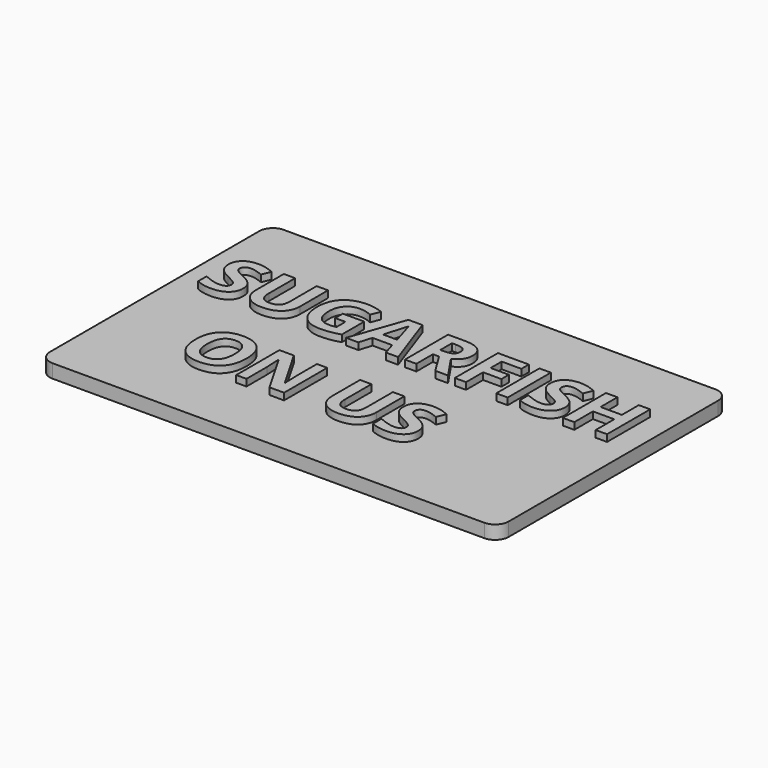
from build123d import *

# Parameters (mm, degrees)
F1_DEPTH     = 2.54
F2_TEXT_SIZE = 14.1111111111
F3_DEPTH     = 1.27


# Not quite as in the source:
# - Text() gives the source's letters only with a copy of the font that has no kerning and outlines rounded to 1/6400 em; it was checked with that copy


with BuildPart() as f1:
    # F0 (on Top) → F1 (new body)
    with BuildSketch(Plane.XY):
        with BuildLine():
            ThreePointArc((42.8625, 24.4475), (42.1185512242, 26.2435512242), (40.3225, 26.9875))
            Line((40.3225, 26.9875), (-40.3225, 26.9875))
            ThreePointArc((-40.3225, 26.9875), (-42.1185512242, 26.2435512242), (-42.8625, 24.4475))
            Line((-42.8625, 24.4475), (-42.8625, -24.4475))
            ThreePointArc((-42.8625, -24.4475), (-42.1185512242, -26.2435512242), (-40.3225, -26.9875))
            Line((-40.3225, -26.9875), (40.3225, -26.9875))
            ThreePointArc((40.3225, -26.9875), (42.1185512242, -26.2435512242), (42.8625, -24.4475))
            Line((42.8625, -24.4475), (42.8625, 24.4475))
        make_face()
    extrude(amount=F1_DEPTH)

    # F2 (on face) → F3 (join)
    with BuildSketch(Plane.XY.offset(2.54)):
        with Locations((-39.0525, 4.1275)):
            Text('SUGARFISH', F2_TEXT_SIZE, font='Open Sans', font_style=FontStyle.BOLD, text_align=(TextAlign.LEFT, TextAlign.BOTTOM))
        with Locations((-28.0524479167, -15.0636111111)):
            Text('ON US', F2_TEXT_SIZE, font='Open Sans', font_style=FontStyle.BOLD, text_align=(TextAlign.LEFT, TextAlign.BOTTOM))
    extrude(amount=F3_DEPTH)


solid = f1.part
